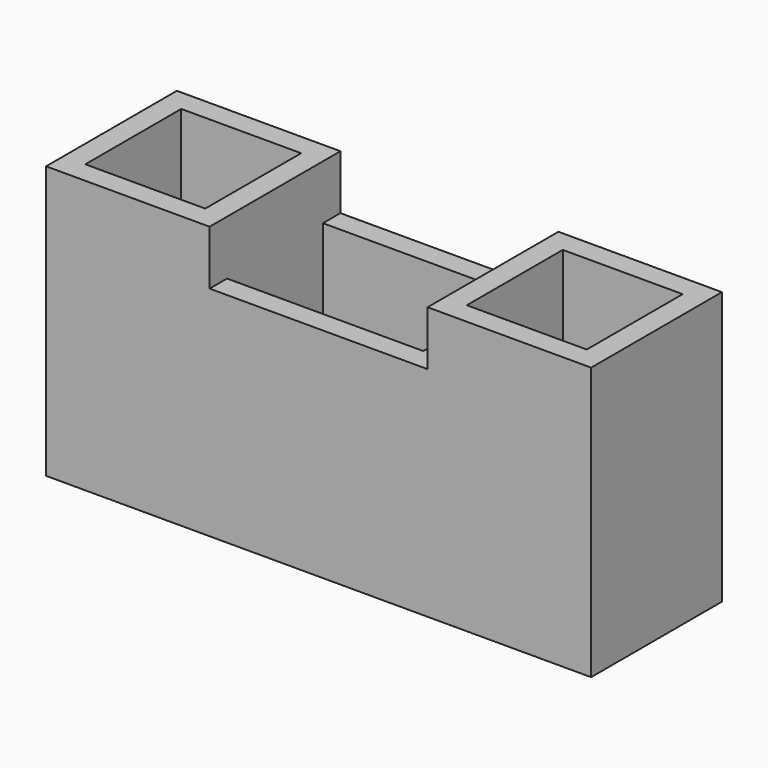
from build123d import *

# Parameters (mm, degrees)
F0_W      = 38.1
F0_H      = 38.1
F1_DEPTH  = 63.5
F2_T      = -5.08
F0_W_2    = 50.8
F3_DEPTH  = 50.8
F0_W_3    = 33.02
F4_DEPTH  = 63.5
F5_T      = -5.08
F0_W_4    = 5.08
F7_DEPTH  = 63.5
F8_DEPTH  = 63.5
F9_T      = -5.08
F10_DEPTH = 50.8


# Not quite as in the source:
# - a shell that OpenCascade refuses in one call is made with other operations: the cavity is built on its own and cut out


with BuildPart() as f1:
    # F0 (on Top) → F1 (new body)
    with BuildSketch(Plane.XY):
        with Locations((-44.45, 0)):
            Rectangle(F0_W, F0_H)
    extrude(amount=F1_DEPTH)

    # F2
    f2_openings = [f1.faces().sort_by_distance(p)[0] for p in [
        (-44.45, 0, 63.5),
    ]]
    offset(amount=F2_T, openings=f2_openings)

    # F0 (on Top) → F3 (join)
    with BuildSketch(Plane.XY):
        Rectangle(F0_W_2, F0_H)
    extrude(amount=F3_DEPTH)

    # F5: a shell. OpenCascade refuses it in one call, so the cavity is built on its own and cut out:
    # the body offset inwards by the wall thickness, plus a prism from it out through each open face.
    f5_core = offset(f1.part, amount=F5_T, kind=Kind.INTERSECTION, mode=Mode.PRIVATE)
    f5_exits = [f5_core.faces().sort_by_distance(p)[0] for p in [
        (-2.54, 0, 45.72),
    ]]
    add(f5_core, mode=Mode.SUBTRACT)
    extrude(f5_exits, amount=-F5_T, mode=Mode.SUBTRACT)

    # F0 (on Top) → F7 (join)
    with BuildSketch(Plane.XY):
        with Locations((27.94, 0)):
            Rectangle(F0_W_4, F0_H)
    extrude(amount=F7_DEPTH)

    # F0 (on Top) → F8 (join)
    with BuildSketch(Plane.XY):
        with Locations((46.99, 0)):
            Rectangle(F0_W_3, F0_H)
    extrude(amount=F8_DEPTH)

    # F9: a shell. OpenCascade refuses it in one call, so the cavity is built on its own and cut out:
    # the body offset inwards by the wall thickness, plus a prism from it out through each open face.
    f9_core = offset(f1.part, amount=F9_T, kind=Kind.INTERSECTION, mode=Mode.PRIVATE)
    f9_exits = [f9_core.faces().sort_by_distance(p)[0] for p in [
        (44.45, 0, 58.42),
    ]]
    add(f9_core, mode=Mode.SUBTRACT)
    extrude(f9_exits, amount=-F9_T, mode=Mode.SUBTRACT)

    # F0 (on Top) → F10 (join)
    with BuildSketch(Plane.XY):
        with Locations((27.94, 0)):
            Rectangle(F0_W_4, F0_H)
    extrude(amount=F10_DEPTH)


with BuildPart() as f4:
    # F0 (on Top) → F4 (new body)
    with BuildSketch(Plane.XY):
        with Locations((46.99, 0)):
            Rectangle(F0_W_3, F0_H)
    extrude(amount=F4_DEPTH)


solid = f1.part
